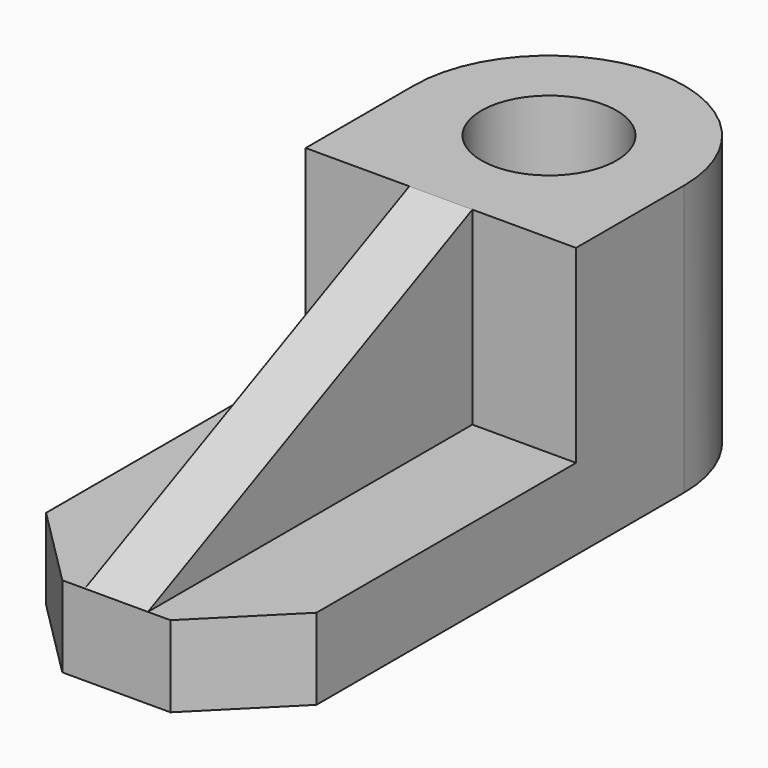
from build123d import *

# Parameters (mm, degrees)
F0_W     = 177.8
F0_H     = 1143
F1_DEPTH = 228.6
F2_DEPTH = 762
F4_DEPTH = 177.8


with BuildPart() as f1:
    # F0 (on Top) → F1 (new body)
    with BuildSketch(Plane.XY):
        Polygon((398.4137039741, -411.6901900116), (398.4137039741, 502.7098099884), (106.3137039741, 502.7098099884), (106.3137039741, -640.2901900116), (169.8137039741, -640.2901900116), align=None)
        with BuildLine():
            Line((398.4137039741, 883.7098099884), (207.9137039741, 883.7098099884))
            ThreePointArc((207.9137039741, 883.7098099884), (17.4137039741, 693.2098099884), (-173.0862960259, 883.7098099884))
            Line((-173.0862960259, 883.7098099884), (-363.5862960259, 883.7098099884))
            Line((-363.5862960259, 883.7098099884), (-363.5862960259, 502.7098099884))
            Line((-363.5862960259, 502.7098099884), (-71.4862960259, 502.7098099884))
            Line((-71.4862960259, 502.7098099884), (106.3137039741, 502.7098099884))
            Line((106.3137039741, 502.7098099884), (398.4137039741, 502.7098099884))
            Line((398.4137039741, 502.7098099884), (398.4137039741, 883.7098099884))
        make_face()
        Polygon((-71.4862960259, 502.7098099884), (-363.5862960259, 502.7098099884), (-363.5862960259, -411.6901900116), (-134.9862960259, -640.2901900116), (-71.4862960259, -640.2901900116), align=None)
        with Locations((17.4137039741, -68.7901900116)):
            Rectangle(F0_W, F0_H)
        with BuildLine():
            ThreePointArc((-173.0862960259, 883.7098099884), (17.4137039741, 1074.2098099884), (207.9137039741, 883.7098099884))
            Line((207.9137039741, 883.7098099884), (398.4137039741, 883.7098099884))
            ThreePointArc((398.4137039741, 883.7098099884), (17.4137039741, 1264.7098099884), (-363.5862960259, 883.7098099884))
            Line((-363.5862960259, 883.7098099884), (-173.0862960259, 883.7098099884))
        make_face()
    extrude(amount=F1_DEPTH)

    # F0 (on Top) → F2 (join)
    with BuildSketch(Plane.XY):
        with BuildLine():
            Line((398.4137039741, 883.7098099884), (207.9137039741, 883.7098099884))
            ThreePointArc((207.9137039741, 883.7098099884), (17.4137039741, 693.2098099884), (-173.0862960259, 883.7098099884))
            Line((-173.0862960259, 883.7098099884), (-363.5862960259, 883.7098099884))
            Line((-363.5862960259, 883.7098099884), (-363.5862960259, 502.7098099884))
            Line((-363.5862960259, 502.7098099884), (-71.4862960259, 502.7098099884))
            Line((-71.4862960259, 502.7098099884), (106.3137039741, 502.7098099884))
            Line((106.3137039741, 502.7098099884), (398.4137039741, 502.7098099884))
            Line((398.4137039741, 502.7098099884), (398.4137039741, 883.7098099884))
        make_face()
        with Locations((17.4137039741, -68.7901900116)):
            Rectangle(F0_W, F0_H)
        with BuildLine():
            ThreePointArc((-173.0862960259, 883.7098099884), (17.4137039741, 1074.2098099884), (207.9137039741, 883.7098099884))
            Line((207.9137039741, 883.7098099884), (398.4137039741, 883.7098099884))
            ThreePointArc((398.4137039741, 883.7098099884), (17.4137039741, 1264.7098099884), (-363.5862960259, 883.7098099884))
            Line((-363.5862960259, 883.7098099884), (-173.0862960259, 883.7098099884))
        make_face()
    extrude(amount=F2_DEPTH)

    # F3 (on face) → F4 (cut)
    with BuildSketch(Plane.YZ.offset(106.3137039741)):
        Polygon((-640.2901900116, 762), (-640.2901900116, 228.6), (502.7098099884, 762), align=None)
    extrude(amount=-F4_DEPTH, mode=Mode.SUBTRACT)


solid = f1.part
